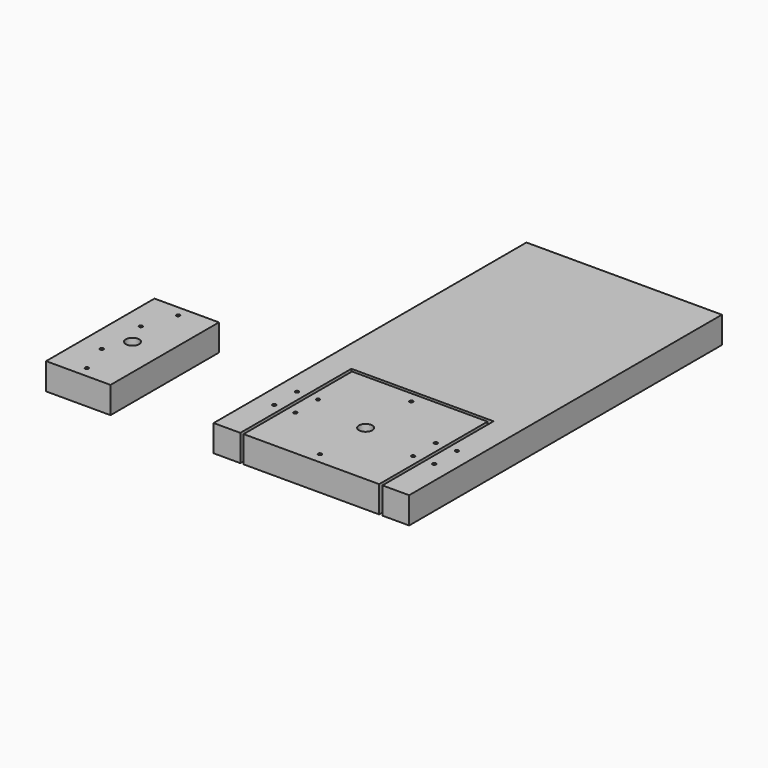
from build123d import *

# Parameters (mm, degrees)
F1_DEPTH = 19.05
F2_D     = 2.4384
F2_2_D   = 2.4384
F3_DEPTH = 19.05
F4_D     = 9.525
F4_2_D   = 9.525
F5_D     = 2.4384


# Not quite as in the source:
# - a feature names something its author has since deleted; it is built from what else it names


with BuildPart() as f1:
    # F0 (on Top) → F1 (new body)
    with BuildSketch(Plane.XY):
        Polygon((50.8, -139.7), (69.85, -139.7), (69.85, 139.7), (-69.85, 139.7), (-69.85, -139.7), (-50.8, -139.7), (-50.8, -40.48125), (50.8, -40.48125), align=None)
    extrude(amount=F1_DEPTH)

    # F2 (through all)
    with Locations(Plane(origin=(0, 0, 0), x_dir=(1, 0, 0), z_dir=(0, 0, -1))):
        with Locations((-57.15, 81.12125), (-57.15, 101.44125), (-42.06875, 101.44125), (-42.06875, 81.12125), (42.06875, 81.12125), (57.15, 81.12125), (57.15, 101.44125), (42.06875, 101.44125), (0, 50.4825), (0, 132.08)):
            Hole(F2_D / 2)


with BuildPart() as f1b:
    # F0 (on Top) → F1, piece 2 (new body)
    with BuildSketch(Plane.XY):
        Polygon((48.41875, -42.8625), (-48.41875, -139.7), (48.41875, -139.7), align=None)
        Polygon((-48.41875, -42.8625), (-48.41875, -139.7), (48.41875, -42.8625), align=None)
    extrude(amount=F1_DEPTH)

    # F2#2 (through all)
    with Locations(Plane(origin=(0, 0, 0), x_dir=(1, 0, 0), z_dir=(0, 0, -1))):
        with Locations((-57.15, 81.12125), (-57.15, 101.44125), (-42.06875, 101.44125), (-42.06875, 81.12125), (42.06875, 81.12125), (57.15, 81.12125), (57.15, 101.44125), (42.06875, 101.44125), (0, 50.4825), (0, 132.08)):
            Hole(F2_2_D / 2)

    # F4 (through all)
    with Locations(Plane(origin=(0, 0, 0), x_dir=(1, 0, 0), z_dir=(0, 0, -1))):
        with Locations((-166.5715282751, 91.28125), (0, 91.28125)):
            Hole(F4_D / 2)


with BuildPart() as f3:
    # F0 (on Top) → F3 (new body)
    with BuildSketch(Plane.XY):
        with BuildLine():
            ThreePointArc((-173.1950164444, -105.2134147701), (-187.2154043393, -85.270226953), (-162.8976236217, -83.5533815912))
            Line((-162.8976236217, -83.5533815912), (-143.5527782751, -42.8625))
            Line((-143.5527782751, -42.8625), (-189.5902782751, -42.8625))
            Line((-189.5902782751, -42.8625), (-189.5902782751, -61.9125))
            Line((-189.5902782751, -61.9125), (-189.5902782751, -120.65))
            Line((-189.5902782751, -120.65), (-189.5902782751, -139.7))
            Line((-189.5902782751, -139.7), (-173.1950164444, -105.2134147701))
        make_face()
        with BuildLine():
            ThreePointArc((-162.8976236217, -83.5533815912), (-161.1656589421, -87.2460712646), (-160.5715282751, -91.28125))
            ThreePointArc((-160.5715282751, -91.28125), (-164.1967712748, -100.6814849537), (-173.1950164444, -105.2134147701))
            Line((-173.1950164444, -105.2134147701), (-189.5902782751, -139.7))
            Line((-189.5902782751, -139.7), (-143.5527782751, -139.7))
            Line((-143.5527782751, -139.7), (-143.5527782751, -83.2121861219))
            Line((-143.5527782751, -83.2121861219), (-143.5527782751, -61.9125))
            Line((-143.5527782751, -61.9125), (-143.5527782751, -42.8625))
            Line((-143.5527782751, -42.8625), (-162.8976236217, -83.5533815912))
        make_face()
        with BuildLine():
            Line((-173.1950164444, -105.2134147701), (-162.8976236217, -83.5533815912))
            ThreePointArc((-162.8976236217, -83.5533815912), (-187.2154043393, -85.270226953), (-173.1950164444, -105.2134147701))
        make_face()
        with BuildLine():
            ThreePointArc((-173.1950164444, -105.2134147701), (-164.1967712748, -100.6814849537), (-160.5715282751, -91.28125))
            ThreePointArc((-160.5715282751, -91.28125), (-161.1656589421, -87.2460712646), (-162.8976236217, -83.5533815912))
            Line((-162.8976236217, -83.5533815912), (-173.1950164444, -105.2134147701))
        make_face()
    extrude(amount=F3_DEPTH)

    # F4#2 (through all)
    with Locations(Plane(origin=(0, 0, 0), x_dir=(1, 0, 0), z_dir=(0, 0, -1))):
        with Locations((-166.5715282751, 91.28125), (0, 91.28125)):
            Hole(F4_2_D / 2)

    # F5 (through all)
    with Locations(Plane(origin=(0, 0, 0), x_dir=(1, 0, 0), z_dir=(0, 0, -1))):
        with Locations((-166.5715282751, 50.4825), (-174.5715282751, 73.78125), (-174.5715282751, 108.78125), (-166.5715282751, 132.08)):
            Hole(F5_D / 2)


solid = Compound([f1.part, f1b.part, f3.part])
